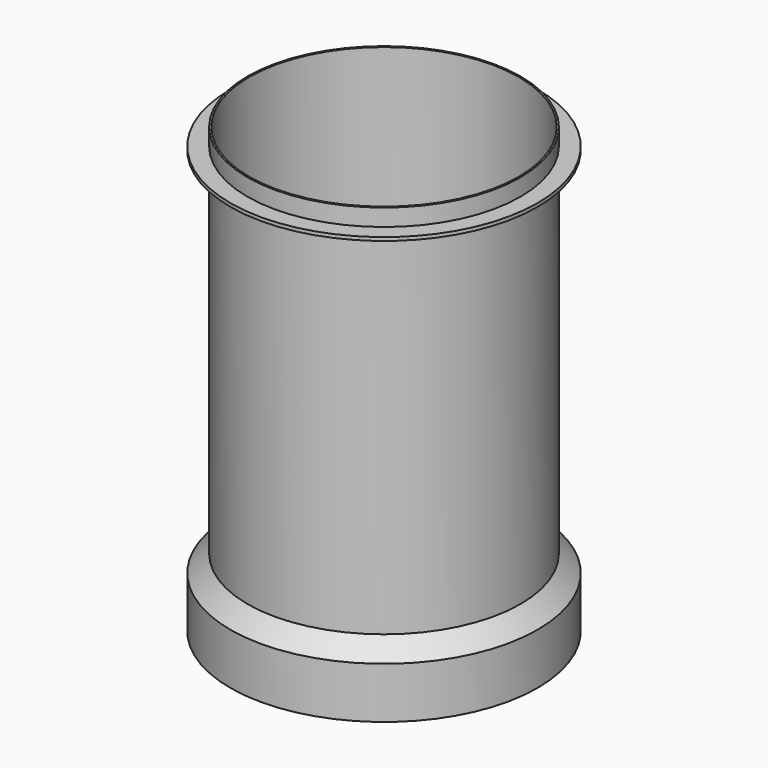
from build123d import *

# Parameters (mm, degrees)
F3_DEPTH = 6.133103


with BuildPart() as f1:
    # F0 (on Front) → F1 (revolve)
    with BuildSketch(Plane.XZ):
        Polygon((0, 5.08), (0, 0), (228.6, 0), (228.6, 76.2), (203.2, 101.6), (203.2, 629.92), (228.6, 629.92), (228.6, 635), (203.2, 635), (203.2, 660.4), (200.66, 660.4), (200.66, 106.68), (191.135, 106.68), (191.135, 101.6), (199.607898, 101.6), (226.06, 75.147898), (226.06, 5.08), align=None)
    revolve(axis=Axis((0, 0, 2.54), (0, 0, -1)))

    # F2 (on face) → F3 (cut, through all)
    with BuildSketch(Plane.XY.offset(106.68)):
        with BuildLine():
            ThreePointArc((-12.7, 200.257698), (-141.888047, 141.888047), (-200.257698, 12.7))
            Line((-200.257698, 12.7), (-190.712606, 12.7))
            ThreePointArc((-190.712606, 12.7), (-135.152855, 135.152855), (-12.7, 190.712606))
            Line((-12.7, 190.712606), (-12.7, 200.257698))
        make_face()
        with BuildLine():
            ThreePointArc((-12.7, -190.712606), (-135.152855, -135.152855), (-190.712606, -12.7))
            Line((-190.712606, -12.7), (-200.257698, -12.7))
            ThreePointArc((-200.257698, -12.7), (-141.888047, -141.888047), (-12.7, -200.257698))
            Line((-12.7, -200.257698), (-12.7, -190.712606))
        make_face()
        with BuildLine():
            ThreePointArc((190.712606, -12.7), (135.152855, -135.152855), (12.7, -190.712606))
            Line((12.7, -190.712606), (12.7, -200.257698))
            ThreePointArc((12.7, -200.257698), (141.888047, -141.888047), (200.257698, -12.7))
            Line((200.257698, -12.7), (190.712606, -12.7))
        make_face()
        with BuildLine():
            ThreePointArc((12.7, 190.712606), (135.152855, 135.152855), (190.712606, 12.7))
            Line((190.712606, 12.7), (200.257698, 12.7))
            ThreePointArc((200.257698, 12.7), (141.888047, 141.888047), (12.7, 200.257698))
            Line((12.7, 200.257698), (12.7, 190.712606))
        make_face()
    extrude(amount=-F3_DEPTH, mode=Mode.SUBTRACT)


solid = f1.part
